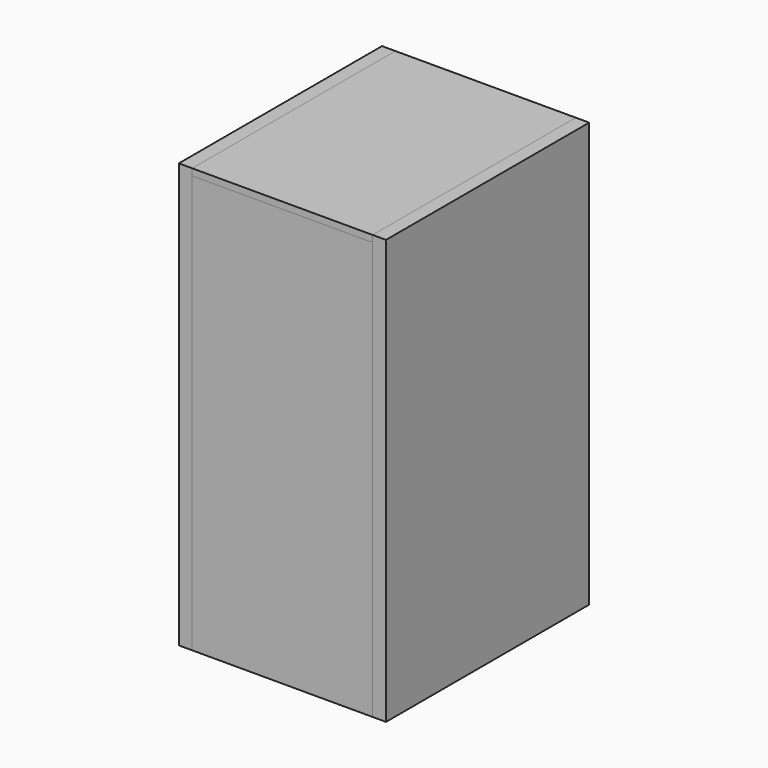
from build123d import *

# Parameters (mm, degrees)
F1_W     = 25.4
F1_H     = 806.45
F2_DEPTH = 482.6
F3_W     = 342.9
F3_H     = 12.7
F4_DEPTH = 482.6
F5_W     = 342.9
F5_H     = 12.7
F6_DEPTH = 793.75
F7_W     = 342.9
F7_H     = 12.7
F8_DEPTH = 793.75


# Not quite as in the source:
# - a feature of the source that left no trace in its solid (it failed there, or was rolled back) is left out


with BuildPart() as f2:
    # F1 (on face) → F2 (new body)
    with BuildSketch(Plane.XZ):
        with Locations((-92.4449153244, 139.9926033994)):
            Rectangle(F1_W, F1_H)
    extrude(amount=F2_DEPTH)


with BuildPart() as f2b:
    # F1 (on face) → F2, piece 2 (new body)
    with BuildSketch(Plane.XZ):
        with Locations((275.8550846756, 139.9926033994)):
            Rectangle(F1_W, F1_H)
    extrude(amount=F2_DEPTH)


with BuildPart() as f4:
    # F3 (on face) → F4 (new body, through all)
    with BuildSketch(Plane.XZ.offset(482.6)):
        with Locations((91.7050846756, 536.8676033994)):
            Rectangle(F3_W, F3_H)
    extrude(amount=-F4_DEPTH)


with BuildPart() as f6:
    # F5 (on face) → F6 (new body, through all)
    with BuildSketch(Plane(origin=(0, 0, -263.2323966006), x_dir=(1, 0, 0), z_dir=(0, 0, -1))):
        with Locations((91.7050846756, 6.35)):
            Rectangle(F5_W, F5_H)
    extrude(amount=-F6_DEPTH)


with BuildPart() as f8:
    # F7 (on face) → F8 (new body, through all)
    with BuildSketch(Plane(origin=(0, 0, 530.5176033994), x_dir=(1, 0, 0), z_dir=(0, 0, -1))):
        with Locations((91.7050846756, 476.25)):
            Rectangle(F7_W, F7_H)
    extrude(amount=F8_DEPTH)


solid = Compound([f2.part, f2b.part, f4.part, f6.part, f8.part])
